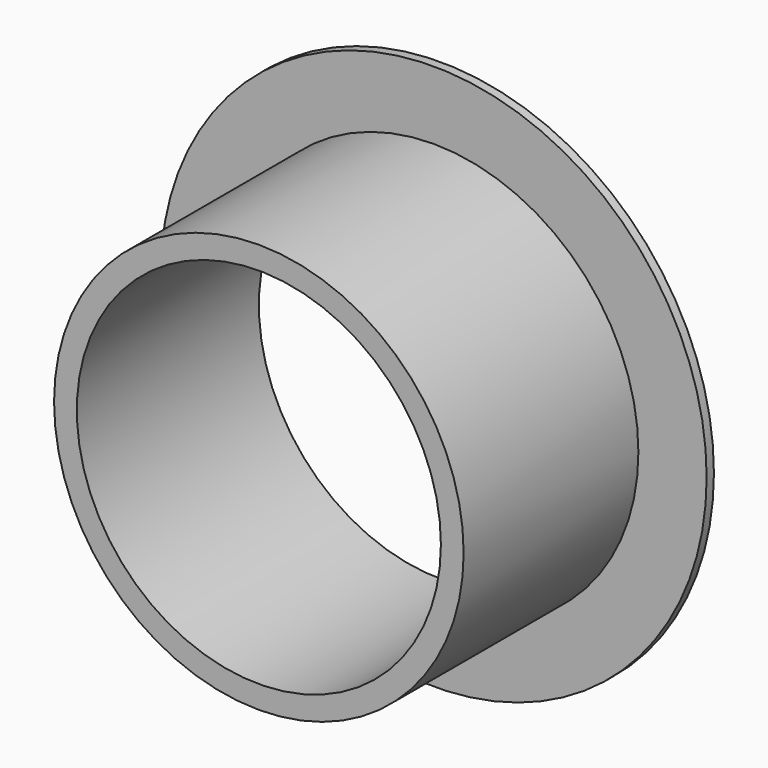
from build123d import *

# Parameters (mm, degrees)
F0_R     = 30
F1_DEPTH = 1
F2_R     = 22.5
F3_DEPTH = 24
F5_R     = 20
F6_DEPTH = 25.001


# Not quite as in the source:
# - the program builds the solid bodies; features that only make, move or delete a surface that nothing else refers to are left out


with BuildPart() as f1:
    # F0 (on Front) → F1 (new body)
    with BuildSketch(Plane.XZ):
        Circle(F0_R)
    extrude(amount=F1_DEPTH)

    # F2 (on face) → F3 (join)
    with BuildSketch(Plane.XZ.offset(1)):
        Circle(F2_R)
    extrude(amount=F3_DEPTH)

    # F5 (on face) → F6 (cut, through all)
    with BuildSketch(Plane.XZ.offset(25)):
        Circle(F5_R)
    extrude(amount=-F6_DEPTH, mode=Mode.SUBTRACT)


solid = f1.part
